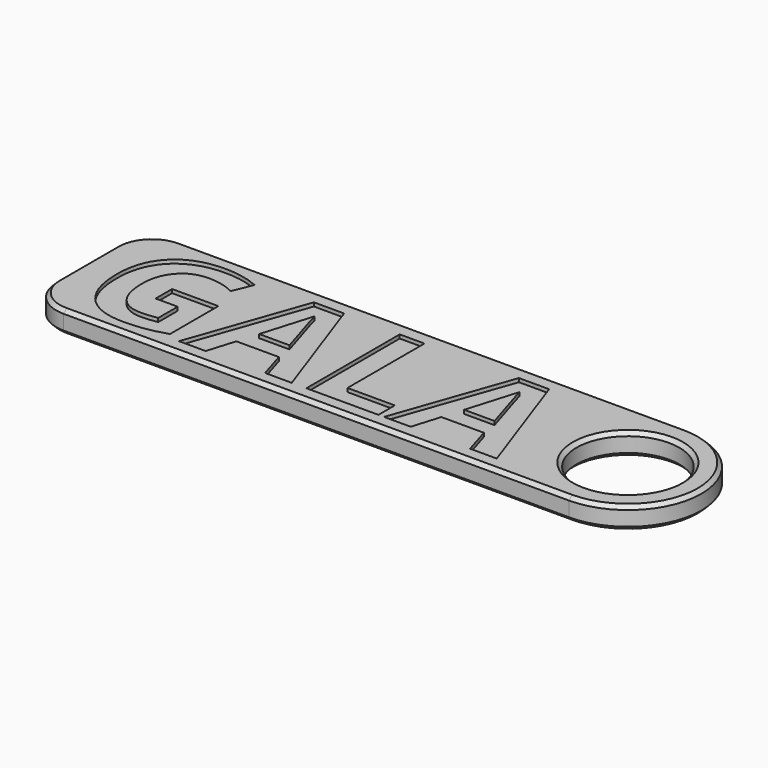
from build123d import *

# Parameters (mm, degrees)
F0_R         = 7
F0_TEXT_SIZE = 22.2222222222
F1_DEPTH     = 3
F2_TEXT_SIZE = 22.2222222222
F3_DEPTH     = 0.5
F4_ANGLE     = 180
F5_DEPTH     = 0.5
F6_SIZE      = 0.5


# Not quite as in the source:
# - Text() gives the source's letters only with a copy of the font that has no kerning and outlines rounded to 1/6400 em; it was checked with that copy


with BuildPart() as f1:
    # F0 (on Top) → F1 (new body)
    with BuildSketch(Plane.XY):
        with BuildLine():
            Line((-68.7534722222, -10), (0, -10))
            ThreePointArc((0, -10), (10, 0), (0, 10))
            Line((0, 10), (-68.7534722222, 10))
            ThreePointArc((-68.7534722222, 10), (-72.2890061282, 8.5355339059), (-73.7534722222, 5))
            Line((-73.7534722222, 5), (-73.7534722222, -5))
            ThreePointArc((-73.7534722222, -5), (-72.2890061282, -8.5355339059), (-68.7534722222, -10))
        make_face()
        with BuildLine():
            Line((-62.7361111111, -1.8923611111), (-62.7361111111, 0.9097222222))
            Line((-62.7361111111, 0.9097222222), (-56.4409722222, 0.9097222222))
            Line((-56.4409722222, 0.9097222222), (-56.4409722222, -7.3159722222))
            add(Edge.make_bspline(
                [(-56.4409722222, -7.3159722222), (-57.9722222222, -7.8159722222), (-59.3229166667, -8.0173611111)],
                knots=[0, 0, 0, 1, 1, 1], degree=2))
            add(Edge.make_bspline(
                [(-59.3229166667, -8.0173611111), (-60.6736111111, -8.21875), (-62.0833333333, -8.21875)],
                knots=[0, 0, 0, 1, 1, 1], degree=2))
            add(Edge.make_bspline(
                [(-62.0833333333, -8.21875), (-65.6736111111, -8.21875), (-67.5677083333, -6.1076388889)],
                knots=[0, 0, 0, 1, 1, 1], degree=2))
            add(Edge.make_bspline(
                [(-67.5677083333, -6.1076388889), (-69.4618055556, -3.9965277778), (-69.4618055556, -0.0451388889)],
                knots=[0, 0, 0, 1, 1, 1], degree=2))
            add(Edge.make_bspline(
                [(-69.4618055556, -0.0451388889), (-69.4618055556, 3.7951388889), (-67.2638888889, 5.9427083333)],
                knots=[0, 0, 0, 1, 1, 1], degree=2))
            add(Edge.make_bspline(
                [(-67.2638888889, 5.9427083333), (-65.0659722222, 8.0902777778), (-61.1736111111, 8.0902777778)],
                knots=[0, 0, 0, 1, 1, 1], degree=2))
            add(Edge.make_bspline(
                [(-61.1736111111, 8.0902777778), (-58.7291666667, 8.0902777778), (-56.4618055556, 7.1145833333)],
                knots=[0, 0, 0, 1, 1, 1], degree=2))
            Line((-56.4618055556, 7.1145833333), (-57.5798611111, 4.4236111111))
            add(Edge.make_bspline(
                [(-57.5798611111, 4.4236111111), (-59.3159722222, 5.2916666667), (-61.1944444444, 5.2916666667)],
                knots=[0, 0, 0, 1, 1, 1], degree=2))
            add(Edge.make_bspline(
                [(-61.1944444444, 5.2916666667), (-63.375, 5.2916666667), (-64.6875, 3.8263888889)],
                knots=[0, 0, 0, 1, 1, 1], degree=2))
            add(Edge.make_bspline(
                [(-64.6875, 3.8263888889), (-66, 2.3611111111), (-66, -0.1111111111)],
                knots=[0, 0, 0, 1, 1, 1], degree=2))
            add(Edge.make_bspline(
                [(-66, -0.1111111111), (-66, -2.6944444444), (-64.9427083333, -4.0555555556)],
                knots=[0, 0, 0, 1, 1, 1], degree=2))
            add(Edge.make_bspline(
                [(-64.9427083333, -4.0555555556), (-63.8854166667, -5.4166666667), (-61.8680555556, -5.4166666667)],
                knots=[0, 0, 0, 1, 1, 1], degree=2))
            add(Edge.make_bspline(
                [(-61.8680555556, -5.4166666667), (-60.8125, -5.4166666667), (-59.7291666667, -5.2013888889)],
                knots=[0, 0, 0, 1, 1, 1], degree=2))
            Line((-59.7291666667, -5.2013888889), (-59.7291666667, -1.8923611111))
            Line((-59.7291666667, -1.8923611111), (-62.7361111111, -1.8923611111))
        make_face(mode=Mode.SUBTRACT)
        Polygon((-39.3298611111, -8), (-42.9548611111, -8), (-44.1041666667, -4.2222222222), (-49.8888888889, -4.2222222222), (-51.0381944444, -8), (-54.6631944444, -8), (-49.0625, 7.9305555556), (-44.9513888889, 7.9305555556), align=None, mode=Mode.SUBTRACT)
        Polygon((-27.5347222222, -8), (-37.3333333333, -8), (-37.3333333333, 7.8645833333), (-33.96875, 7.8645833333), (-33.96875, -5.2222222222), (-27.5347222222, -5.2222222222), align=None, mode=Mode.SUBTRACT)
        Polygon((-11.4409722222, -8), (-15.0659722222, -8), (-16.2152777778, -4.2222222222), (-22, -4.2222222222), (-23.1493055556, -8), (-26.7743055556, -8), (-21.1736111111, 7.9305555556), (-17.0625, 7.9305555556), align=None, mode=Mode.SUBTRACT)
        Circle(F0_R, mode=Mode.SUBTRACT)
        with BuildLine():
            Line((-21.1527777778, -1.4027777778), (-17.0208333333, -1.4027777778))
            add(Edge.make_bspline(
                [(-17.0208333333, -1.4027777778), (-18.6145833333, 3.7291666667), (-18.8159722222, 4.4027777778)],
                knots=[0, 0, 0, 1, 1, 1], degree=2))
            add(Edge.make_bspline(
                [(-18.8159722222, 4.4027777778), (-19.0173611111, 5.0763888889), (-19.1041666667, 5.4652777778)],
                knots=[0, 0, 0, 1, 1, 1], degree=2))
            add(Edge.make_bspline(
                [(-19.1041666667, 5.4652777778), (-19.4618055556, 4.0763888889), (-21.1527777778, -1.4027777778)],
                knots=[0, 0, 0, 1, 1, 1], degree=2))
        make_face()
        with BuildLine():
            Line((-49.0416666667, -1.4027777778), (-44.9097222222, -1.4027777778))
            add(Edge.make_bspline(
                [(-44.9097222222, -1.4027777778), (-46.5034722222, 3.7291666667), (-46.7048611111, 4.4027777778)],
                knots=[0, 0, 0, 1, 1, 1], degree=2))
            add(Edge.make_bspline(
                [(-46.7048611111, 4.4027777778), (-46.90625, 5.0763888889), (-46.9930555556, 5.4652777778)],
                knots=[0, 0, 0, 1, 1, 1], degree=2))
            add(Edge.make_bspline(
                [(-46.9930555556, 5.4652777778), (-47.3506944444, 4.0763888889), (-49.0416666667, -1.4027777778)],
                knots=[0, 0, 0, 1, 1, 1], degree=2))
        make_face()
        with Locations((-70.7534722222, -8)):
            Text('GALA', F0_TEXT_SIZE, font='Open Sans', font_style=FontStyle.BOLD, text_align=(TextAlign.LEFT, TextAlign.BOTTOM))
    extrude(amount=F1_DEPTH)

    # F2 (on face) → F3 (cut)
    with BuildSketch(Plane.XY.offset(3)):
        with Locations((-70.7534722222, -8)):
            Text('GALA', F2_TEXT_SIZE, font='Open Sans', font_style=FontStyle.BOLD, text_align=(TextAlign.LEFT, TextAlign.BOTTOM))
    extrude(amount=-F3_DEPTH, mode=Mode.SUBTRACT)


with BuildPart() as f1_1:
    # F4: moved
    add(f1.part.rotate(Axis((-8.5, 0, 0), (1, 0, 0)), F4_ANGLE))

    # F0 (on Top) → F5 (cut)
    with BuildSketch(Plane.XY):
        with Locations((-70.7534722222, -8)):
            Text('GALA', F0_TEXT_SIZE, font='Open Sans', font_style=FontStyle.BOLD, text_align=(TextAlign.LEFT, TextAlign.BOTTOM))
    extrude(amount=-F5_DEPTH, mode=Mode.SUBTRACT)

    # F6
    f6_edges = [f1_1.edges().sort_by_distance(p)[0] for p in [
        (-34.376736, -10, 0),
        (-7, 0, 0),
        (10, 0, -3),
        (-7, 0, -3),
    ]]
    chamfer(f6_edges, length=F6_SIZE)


solid = f1_1.part
